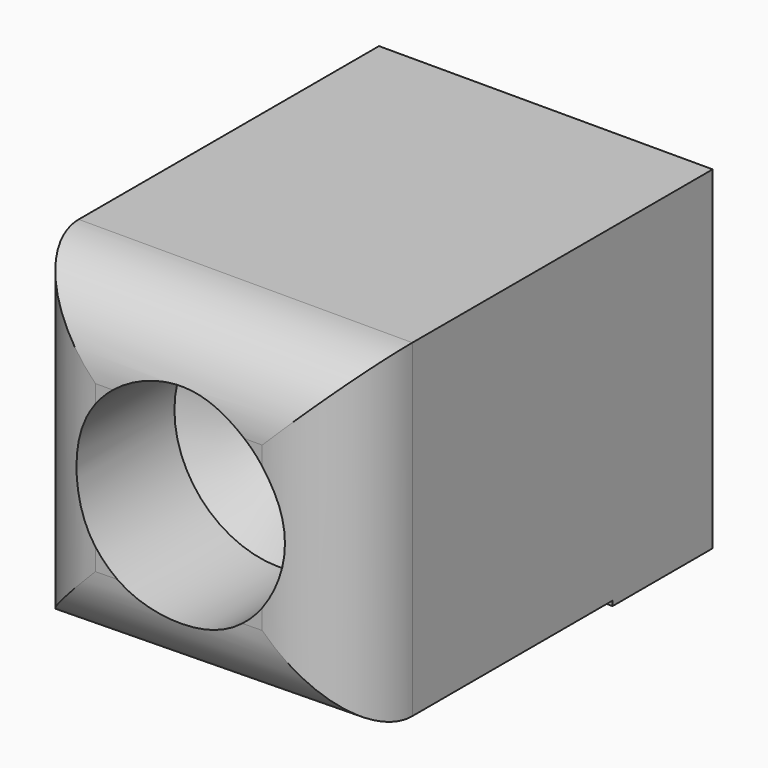
from build123d import *

# Parameters (mm, degrees)
F0_W        = 20.32
F0_H        = 20.32
F1_DEPTH    = 7.62
F3_DEPTH    = 20.32
F5_D        = 12.7
F5_DEPTH    = 7.62
F5_TIP      = 3.8154649308
F6_T1_DEPTH = 45.72
F6_T3_DEPTH = 45.4214045093
F6_T5_DEPTH = 45.72
F6_T7_DEPTH = 45.7221937612


# Not quite as in the source:
# - a fillet or chamfer that OpenCascade refuses, or shapes differently, is made with other operations: its cross-section is extruded or revolved along the edge and cut away or added


with BuildPart() as f1:
    # F0 (on Front) → F1 (new body)
    with BuildSketch(Plane.XZ):
        with Locations((-2.1305914207, -0.150394626)):
            Rectangle(F0_W, F0_H)
    extrude(amount=F1_DEPTH)

    # F2 (on face) → F3 (join)
    with BuildSketch(Plane.XZ.offset(7.62)):
        Polygon((-12.2905914207, 10.009605374), (-12.2905914207, -10.310394626), (8.0294085793, -10.0117991352), (8.0294085793, 10.009605374), align=None)
    extrude(amount=F3_DEPTH)

    # F5
    with Locations(Plane.XZ.offset(27.94)):
        with Locations((-2.1422964055, 0)):
            Hole(F5_D / 2, depth=F5_DEPTH)
            with Locations((0, 0, -(F5_DEPTH + F5_TIP / 2))):  # 118° drill point
                Cone(0, F5_D / 2, F5_TIP, mode=Mode.SUBTRACT)

    # F6: fillet of radius 5.08 on 4 edges, made by hand

    # F6_s2 → F6_t1 (cut)
    with BuildSketch(Plane.YZ.offset(-24.9905914207)):
        with BuildLine():
            ThreePointArc((-22.86, 10.009605374), (-26.4521024484, 8.5217078225), (-27.94, 4.929605374))
            Line((-27.94, 4.929605374), (-27.94, 10.009605374))
            Line((-27.94, 10.009605374), (-22.86, 10.009605374))
        make_face()
    extrude(amount=F6_T1_DEPTH, mode=Mode.SUBTRACT)

    # F6_s4 → F6_t3 (cut)
    with BuildSketch(Plane.XY.offset(-22.7117991352)):
        with BuildLine():
            ThreePointArc((8.0294085793, -22.86), (6.5415110277, -26.4521024484), (2.9494085793, -27.94))
            Line((2.9494085793, -27.94), (8.0294085793, -27.94))
            Line((8.0294085793, -27.94), (8.0294085793, -22.86))
        make_face()
    extrude(amount=F6_T3_DEPTH, mode=Mode.SUBTRACT)

    # F6_s6 → F6_t5 (cut)
    with BuildSketch(Plane.XY.offset(-23.010394626)):
        with BuildLine():
            ThreePointArc((-7.2105914207, -27.94), (-10.8026938691, -26.4521024484), (-12.2905914207, -22.86))
            Line((-12.2905914207, -22.86), (-12.2905914207, -27.94))
            Line((-12.2905914207, -27.94), (-7.2105914207, -27.94))
        make_face()
    extrude(amount=F6_T5_DEPTH, mode=Mode.SUBTRACT)

    # F6_s8 → F6_t7 (cut)
    with BuildSketch(Plane(origin=(-25.138042131, 0, -0.3693949816), x_dir=(0, 1, 0), z_dir=(0.999892051, 0, 0.0146930737))):
        with BuildLine():
            ThreePointArc((-27.94, -5.0486950632), (-26.4521024484, -8.6407975117), (-22.86, -10.1286950632))
            Line((-22.86, -10.1286950632), (-27.94, -10.1286950632))
            Line((-27.94, -10.1286950632), (-27.94, -5.0486950632))
        make_face()
    extrude(amount=F6_T7_DEPTH, mode=Mode.SUBTRACT)


solid = f1.part
